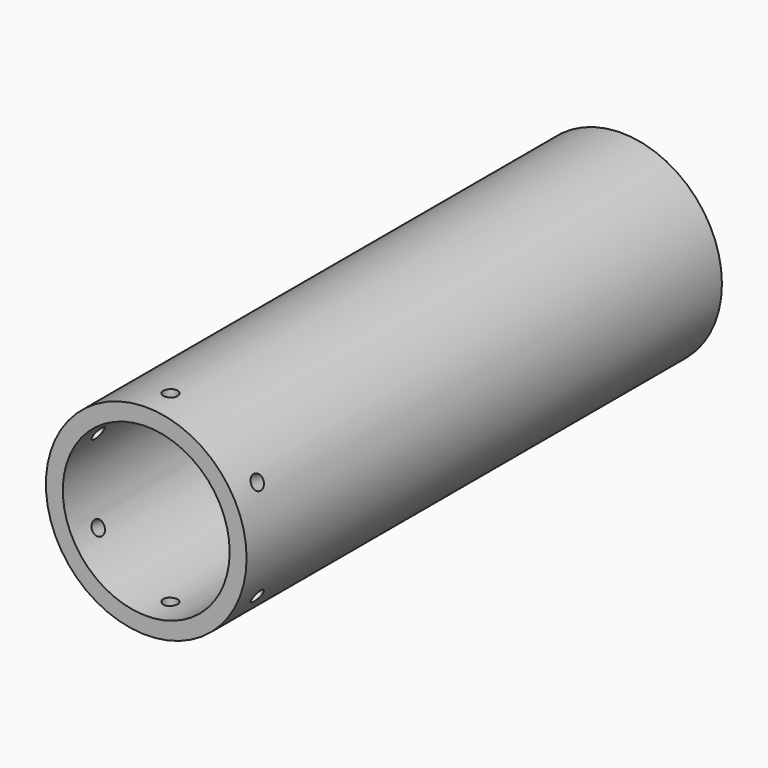
from build123d import *

# Parameters (mm, degrees)
F0_R            = 21.082
F0_R_2          = 17.526
F1_DEPTH        = 124.8156
F2_R            = 1.5
F3_DEPTH        = 25.4
F3_COPIES_COUNT = 6


# Not quite as in the source:
# - a pattern or mirror of a feature is missing from the dataset's text; its kind, count and spacing are read off the source's solid


with BuildPart() as f1:
    # F0 (on Front) → F1 (new body)
    with BuildSketch(Plane.XZ):
        Circle(F0_R)
        Circle(F0_R_2, mode=Mode.SUBTRACT)
    extrude(amount=F1_DEPTH)

    # F2 (on Top) → F3 (cut)
    with BuildSketch(Plane.XY):
        with Locations((0, -118.4656)):
            Circle(F2_R)
    f3 = extrude(amount=F3_DEPTH, mode=Mode.SUBTRACT)

    # F3_copies: F3 ×6 about axis
    f3_copies_axis = Axis((0, 0, 0), (0, 1, 0))
    for i in range(1, F3_COPIES_COUNT):
        add(f3.rotate(f3_copies_axis, i * 360 / F3_COPIES_COUNT), mode=Mode.SUBTRACT)


solid = f1.part
